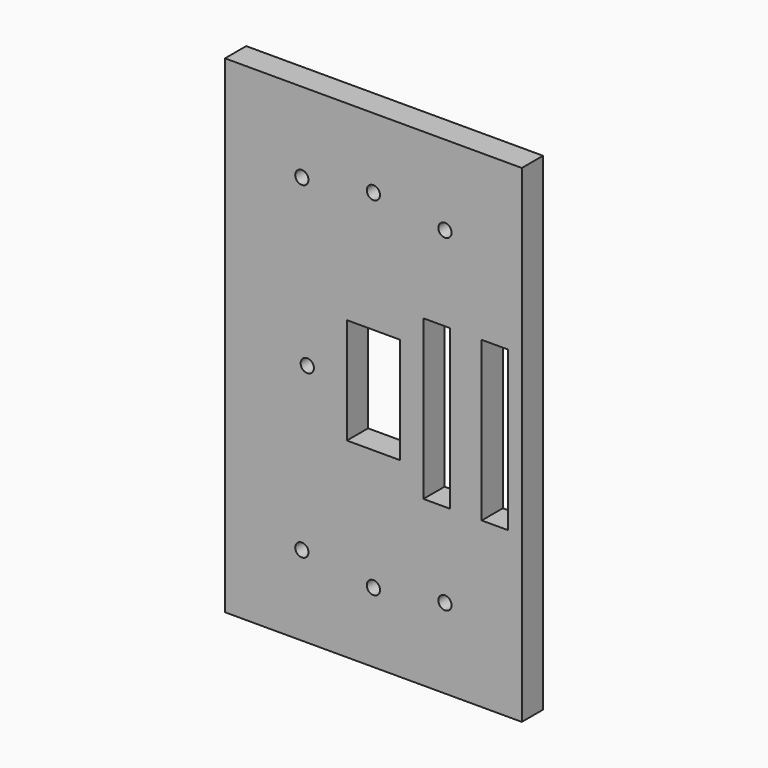
from build123d import *

# Parameters (mm, degrees)
F0_R     = 1.5875
F0_W     = 6.35
F0_H     = 38.1
F1_DEPTH = 3.175
F2_DEPTH = 2.54


# Not quite as in the source:
# - a feature names something its author has since deleted; it is built from what else it names


with BuildPart() as f1:
    # F0 (on Front) → F1 (new body, symmetric)
    with BuildSketch(Plane.XZ):
        Polygon((35.56, -58.42), (35.56, 58.42), (-35.56, 58.42), (-35.56, 0), (-35.56, -58.42), align=None)
        with Locations((-17.1425342897, -39.2875)):
            Circle(F0_R, mode=Mode.SUBTRACT)
        with Locations((0, -41.656)):
            Circle(F0_R, mode=Mode.SUBTRACT)
        with BuildLine():
            ThreePointArc((-14.2624473298, 0), (-15.8499473298, -1.5875), (-17.4374473298, 0))
            ThreePointArc((-17.4374473298, 0), (-15.8499473298, 1.5875), (-14.2624473298, 0))
        make_face(mode=Mode.SUBTRACT)
        Polygon((-6.35, -12.7), (-6.35, 12.7), (0, 12.7), (6.35, 12.7), (6.35, -12.7), align=None, mode=Mode.SUBTRACT)
        with Locations((17.1425342897, -39.2875)):
            Circle(F0_R, mode=Mode.SUBTRACT)
        with Locations((15.1556345809, 0)):
            Rectangle(F0_W, F0_H, mode=Mode.SUBTRACT)
        with Locations((29.1256345809, 0)):
            Rectangle(F0_W, F0_H, mode=Mode.SUBTRACT)
        with Locations((-17.1425342897, 39.2875)):
            Circle(F0_R, mode=Mode.SUBTRACT)
        with BuildLine():
            ThreePointArc((1.5875, 41.656), (1.1225320151, 40.5334679849), (0, 40.0685))
            ThreePointArc((0, 40.0685), (-1.1225320151, 42.7785320151), (1.5875, 41.656))
        make_face(mode=Mode.SUBTRACT)
        with Locations((17.1425342897, 39.2875)):
            Circle(F0_R, mode=Mode.SUBTRACT)
    extrude(amount=F1_DEPTH, both=True)

    # F0 (on Front) → F2 (cut)
    with BuildSketch(Plane.XZ):
        with Locations((15.1556345809, 0)):
            Rectangle(F0_W, F0_H)
        with Locations((29.1256345809, 0)):
            Rectangle(F0_W, F0_H)
    extrude(amount=-F2_DEPTH, mode=Mode.SUBTRACT)


solid = f1.part
